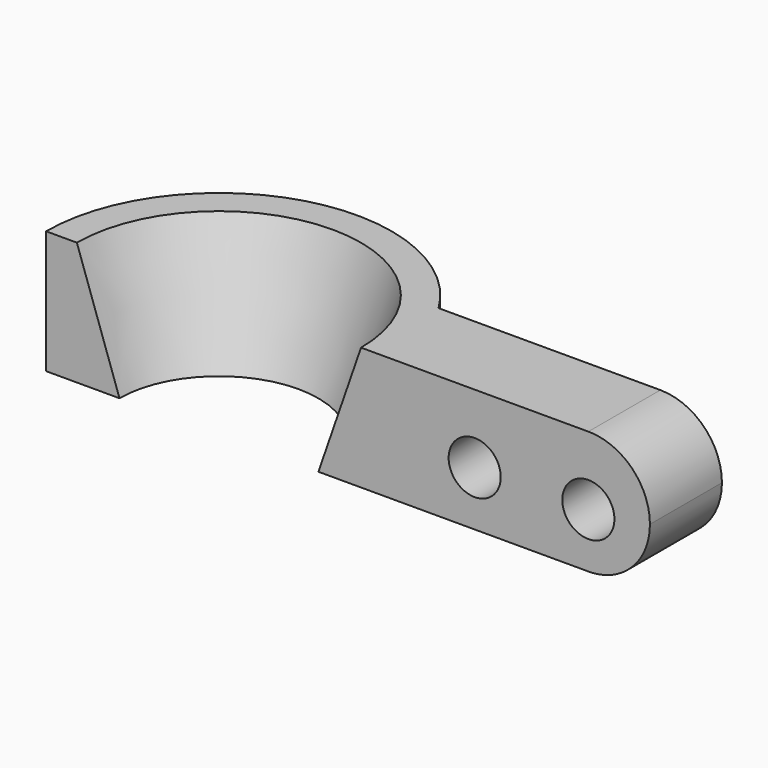
from build123d import *

# Parameters (mm, degrees)
F4_R     = 25.999
F5_R     = 11
F6_DEPTH = 73.0010001


# Not quite as in the source:
# - a fillet or chamfer is up to 0.001 mm smaller than in the source, because OpenCascade refuses the exact size


with BuildPart() as f3:
    # F2 (on offset) → F3 section 0
    with BuildSketch(Plane.XY.offset(52)):
        with BuildLine():
            ThreePointArc((-60, 0), (0, 60), (60, 0))
            Line((60, 0), (182, 0))
            Line((182, 0), (182, 38))
            Line((182, 38), (62.329768169, 38))
            ThreePointArc((62.329768169, 38), (-19.7348286497, 70.2818364741), (-73, 0))
            Line((-73, 0), (-60, 0))
        make_face()
    # F0 (on Top) → F3 section 1
    with BuildSketch(Plane.XY):
        with BuildLine():
            ThreePointArc((-42, 0), (0, 42), (42, 0))
            Line((42, 0), (182, 0))
            Line((182, 0), (182, 38))
            Line((182, 38), (62.329768169, 38))
            ThreePointArc((62.329768169, 38), (-19.7348286497, 70.2818364741), (-73, 0))
            Line((-73, 0), (-42, 0))
        make_face()
    loft()

    # F4 (radius 26 in the source; OpenCascade refuses exactly that, so slightly less here)
    f4_edges = [f3.edges().sort_by_distance(p)[0] for p in [
        (182, 19, 52),
        (182, 19, 0),
    ]]
    fillet(f4_edges, radius=F4_R)

    # F5 (on face) → F6 (cut, through all)
    with BuildSketch(Plane.XZ):
        with Locations((108, 23.0308622122)):
            Circle(F5_R)
        with Locations((156, 23.0308622122)):
            Circle(F5_R)
    extrude(amount=-F6_DEPTH, mode=Mode.SUBTRACT)


solid = f3.part
